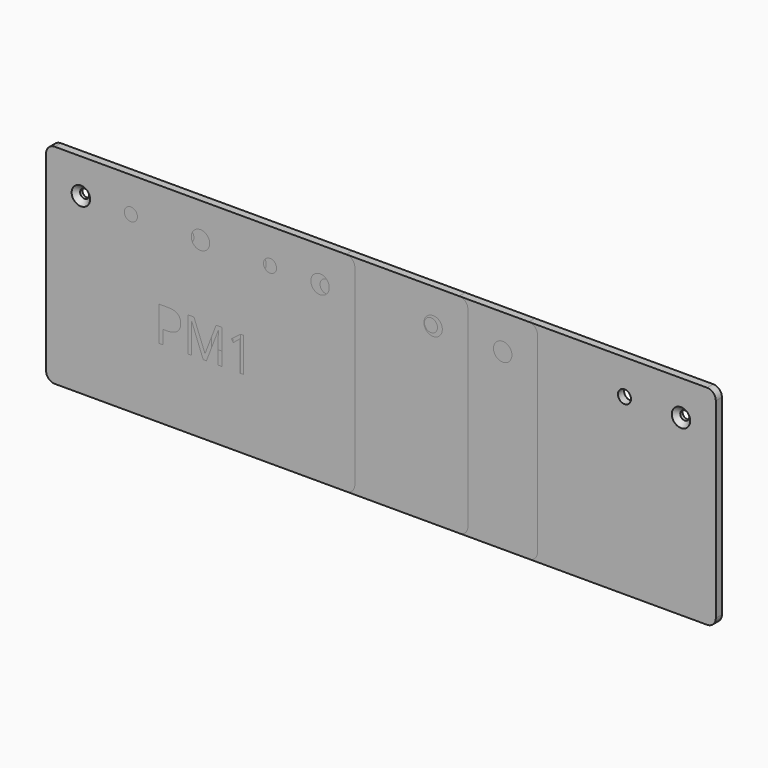
from build123d import *

# Parameters (mm, degrees)
F1_W            = 488.95
F1_H            = 152.4
F2_DEPTH        = 5.588
F3_D            = 9.525
F4_D            = 6.6
F4_CSINK_D      = 13.44
F4_CSINK_ANGLE  = 90
F5_R            = 6.35
F6_W            = 358.775
F6_H            = 152.4
F7_DEPTH        = 5.588
F8_R            = 6.35
F9_D            = 9.525
F10_D           = 6.6
F10_CSINK_D     = 13.44
F10_CSINK_ANGLE = 90
F11_W           = 307.975
F11_H           = 152.4
F12_DEPTH       = 5.588
F13_R           = 6.35
F14_D           = 9.525
F15_D           = 6.6
F15_CSINK_D     = 13.44
F15_CSINK_ANGLE = 90
F16_W           = 225.425
F16_H           = 152.4
F17_DEPTH       = 5.588
F18_R           = 6.35
F19_D           = 6.6
F19_CSINK_D     = 13.44
F19_CSINK_ANGLE = 90
F20_D           = 9.525


# Not quite as in the source:
# - a variable given as a bare number and used for a length is read in inches; the dataset says mm whatever the document's units were
# - a length typed as a fraction of an inch, garbled in the dataset ("3 / 203.2 mm" for 3/8 in), is restored


with BuildPart() as f2:
    # F1 (on Front) → F2 (new body)
    with BuildSketch(Plane.XZ):
        with Locations((244.475, -76.2)):
            Rectangle(F1_W, F1_H)
        with BuildLine():
            add(Edge.make_bspline(
                [(217.0492838542, -76.4149739583), (226.4860894097, -76.4149739583), (226.4860894097, -83.7516493056)],
                knots=[0, 0, 0, 1, 1, 1], degree=2))
            add(Edge.make_bspline(
                [(226.4860894097, -83.7516493056), (226.4860894097, -87.5770833333), (223.8760850694, -89.6358723958)],
                knots=[0, 0, 0, 1, 1, 1], degree=2))
            add(Edge.make_bspline(
                [(223.8760850694, -89.6358723958), (221.2660807292, -91.6946614583), (216.4098741319, -91.6946614583)],
                knots=[0, 0, 0, 1, 1, 1], degree=2))
            Line((216.4098741319, -91.6946614583), (213.4443359375, -91.6946614583))
            Line((213.4443359375, -91.6946614583), (213.4443359375, -101.6))
            Line((213.4443359375, -101.6), (210.5173828125, -101.6))
            Line((210.5173828125, -101.6), (210.5173828125, -76.4149739583))
            Line((210.5173828125, -76.4149739583), (217.0492838542, -76.4149739583))
        make_face(mode=Mode.SUBTRACT)
        with BuildLine():
            Line((245.2604817708, -101.6), (242.9012803819, -101.6))
            Line((242.9012803819, -101.6), (234.3574435764, -79.27578125))
            Line((234.3574435764, -79.27578125), (234.2196397569, -79.27578125))
            add(Edge.make_bspline(
                [(234.2196397569, -79.27578125), (234.4621744792, -81.9271267361), (234.4621744792, -85.5816840278)],
                knots=[0, 0, 0, 1, 1, 1], degree=2))
            Line((234.4621744792, -85.5816840278), (234.4621744792, -101.6))
            Line((234.4621744792, -101.6), (231.7557074653, -101.6))
            Line((231.7557074653, -101.6), (231.7557074653, -76.4149739583))
            Line((231.7557074653, -76.4149739583), (236.1654296875, -76.4149739583))
            Line((236.1654296875, -76.4149739583), (244.1415147569, -97.1902777778))
            Line((244.1415147569, -97.1902777778), (244.2793185764, -97.1902777778))
            Line((244.2793185764, -97.1902777778), (252.3215494792, -76.4149739583))
            Line((252.3215494792, -76.4149739583), (256.6981987847, -76.4149739583))
            Line((256.6981987847, -76.4149739583), (256.6981987847, -101.6))
            Line((256.6981987847, -101.6), (253.7712456597, -101.6))
            Line((253.7712456597, -101.6), (253.7712456597, -85.3722222222))
            add(Edge.make_bspline(
                [(253.7712456597, -85.3722222222), (253.7712456597, -82.5830729167), (254.0137803819, -79.3088541667)],
                knots=[0, 0, 0, 1, 1, 1], degree=2))
            Line((254.0137803819, -79.3088541667), (253.8759765625, -79.3088541667))
            Line((253.8759765625, -79.3088541667), (245.2604817708, -101.6))
        make_face(mode=Mode.SUBTRACT)
        Polygon((279.6067057292, -93.2105034722), (279.6067057292, -95.8122395833), (275.8694661458, -95.8122395833), (275.8694661458, -101.6), (273.1299262153, -101.6), (273.1299262153, -95.8122395833), (260.8819227431, -95.8122395833), (260.8819227431, -93.315234375), (272.8377821181, -76.2771701389), (275.8694661458, -76.2771701389), (275.8694661458, -93.2105034722), align=None, mode=Mode.SUBTRACT)
    extrude(amount=-F2_DEPTH)

    # F3 (through all)
    with Locations(Plane.XZ):
        with Locations((66.675, -25.4), (422.275, -25.4)):
            Hole(F3_D / 2)

    # F4 (through all)
    with Locations(Plane.XZ):
        with Locations((25.4, -25.4), (463.55, -25.4), (311.15, -25.4), (177.8, -25.4)):
            CounterSinkHole(F4_D / 2, F4_CSINK_D / 2, counter_sink_angle=F4_CSINK_ANGLE)

    # F5
    f5_edges = [f2.edges().sort_by_distance(p)[0] for p in [
        (0, 2.794, 0),
        (488.95, 2.794, 0),
        (488.95, 2.794, -152.4),
        (0, 2.794, -152.4),
    ]]
    fillet(f5_edges, radius=F5_R)


with BuildPart() as f7:
    # F6 (on Front) → F7 (new body)
    with BuildSketch(Plane.XZ):
        with Locations((179.3875, -76.2)):
            Rectangle(F6_W, F6_H)
        with BuildLine():
            add(Edge.make_bspline(
                [(152.6425347222, -76.4149739583), (162.0793402778, -76.4149739583), (162.0793402778, -83.7516493056)],
                knots=[0, 0, 0, 1, 1, 1], degree=2))
            add(Edge.make_bspline(
                [(162.0793402778, -83.7516493056), (162.0793402778, -87.5770833333), (159.4693359375, -89.6358723958)],
                knots=[0, 0, 0, 1, 1, 1], degree=2))
            add(Edge.make_bspline(
                [(159.4693359375, -89.6358723958), (156.8593315972, -91.6946614583), (152.003125, -91.6946614583)],
                knots=[0, 0, 0, 1, 1, 1], degree=2))
            Line((152.003125, -91.6946614583), (149.0375868056, -91.6946614583))
            Line((149.0375868056, -91.6946614583), (149.0375868056, -101.6))
            Line((149.0375868056, -101.6), (146.1106336806, -101.6))
            Line((146.1106336806, -101.6), (146.1106336806, -76.4149739583))
            Line((146.1106336806, -76.4149739583), (152.6425347222, -76.4149739583))
        make_face(mode=Mode.SUBTRACT)
        with BuildLine():
            Line((180.8537326389, -101.6), (178.49453125, -101.6))
            Line((178.49453125, -101.6), (169.9506944444, -79.27578125))
            Line((169.9506944444, -79.27578125), (169.812890625, -79.27578125))
            add(Edge.make_bspline(
                [(169.812890625, -79.27578125), (170.0554253472, -81.9271267361), (170.0554253472, -85.5816840278)],
                knots=[0, 0, 0, 1, 1, 1], degree=2))
            Line((170.0554253472, -85.5816840278), (170.0554253472, -101.6))
            Line((170.0554253472, -101.6), (167.3489583333, -101.6))
            Line((167.3489583333, -101.6), (167.3489583333, -76.4149739583))
            Line((167.3489583333, -76.4149739583), (171.7586805556, -76.4149739583))
            Line((171.7586805556, -76.4149739583), (179.734765625, -97.1902777778))
            Line((179.734765625, -97.1902777778), (179.8725694444, -97.1902777778))
            Line((179.8725694444, -97.1902777778), (187.9148003472, -76.4149739583))
            Line((187.9148003472, -76.4149739583), (192.2914496528, -76.4149739583))
            Line((192.2914496528, -76.4149739583), (192.2914496528, -101.6))
            Line((192.2914496528, -101.6), (189.3644965278, -101.6))
            Line((189.3644965278, -101.6), (189.3644965278, -85.3722222222))
            add(Edge.make_bspline(
                [(189.3644965278, -85.3722222222), (189.3644965278, -82.5830729167), (189.60703125, -79.3088541667)],
                knots=[0, 0, 0, 1, 1, 1], degree=2))
            Line((189.60703125, -79.3088541667), (189.4692274306, -79.3088541667))
            Line((189.4692274306, -79.3088541667), (180.8537326389, -101.6))
        make_face(mode=Mode.SUBTRACT)
        with BuildLine():
            add(Edge.make_bspline(
                [(211.0327690972, -77.7351345486), (213.0667534722, -79.4135850694), (213.0667534722, -82.3405381944)],
                knots=[0, 0, 0, 1, 1, 1], degree=2))
            add(Edge.make_bspline(
                [(213.0667534722, -82.3405381944), (213.0667534722, -84.7548611111), (211.7135199653, -86.2872395833)],
                knots=[0, 0, 0, 1, 1, 1], degree=2))
            add(Edge.make_bspline(
                [(211.7135199653, -86.2872395833), (210.3602864583, -87.8196180556), (207.8798177083, -88.3377604167)],
                knots=[0, 0, 0, 1, 1, 1], degree=2))
            Line((207.8798177083, -88.3377604167), (207.8798177083, -88.4755642361))
            add(Edge.make_bspline(
                [(207.8798177083, -88.4755642361), (210.9115017361, -88.850390625), (212.3749782986, -90.4020616319)],
                knots=[0, 0, 0, 1, 1, 1], degree=2))
            add(Edge.make_bspline(
                [(212.3749782986, -90.4020616319), (213.8384548611, -91.9537326389), (213.8384548611, -94.4672743056)],
                knots=[0, 0, 0, 1, 1, 1], degree=2))
            add(Edge.make_bspline(
                [(213.8384548611, -94.4672743056), (213.8384548611, -98.0667100694), (211.3414496528, -100.0069878472)],
                knots=[0, 0, 0, 1, 1, 1], degree=2))
            add(Edge.make_bspline(
                [(211.3414496528, -100.0069878472), (208.8444444444, -101.947265625), (204.2473090278, -101.947265625)],
                knots=[0, 0, 0, 1, 1, 1], degree=2))
            add(Edge.make_bspline(
                [(204.2473090278, -101.947265625), (202.2463975694, -101.947265625), (200.5844835069, -101.6440972222)],
                knots=[0, 0, 0, 1, 1, 1], degree=2))
            add(Edge.make_bspline(
                [(200.5844835069, -101.6440972222), (198.9225694444, -101.3409288194), (197.3571180556, -100.5857638889)],
                knots=[0, 0, 0, 1, 1, 1], degree=2))
            Line((197.3571180556, -100.5857638889), (197.3571180556, -97.8627604167))
            add(Edge.make_bspline(
                [(197.3571180556, -97.8627604167), (198.9942274306, -98.673046875), (200.8463107639, -99.0947265625)],
                knots=[0, 0, 0, 1, 1, 1], degree=2))
            add(Edge.make_bspline(
                [(200.8463107639, -99.0947265625), (202.6983940972, -99.51640625), (204.3520399306, -99.51640625)],
                knots=[0, 0, 0, 1, 1, 1], degree=2))
            add(Edge.make_bspline(
                [(204.3520399306, -99.51640625), (210.8784288194, -99.51640625), (210.8784288194, -94.4011284722)],
                knots=[0, 0, 0, 1, 1, 1], degree=2))
            add(Edge.make_bspline(
                [(210.8784288194, -94.4011284722), (210.8784288194, -89.8150173611), (203.6795572917, -89.8150173611)],
                knots=[0, 0, 0, 1, 1, 1], degree=2))
            Line((203.6795572917, -89.8150173611), (201.1990885417, -89.8150173611))
            Line((201.1990885417, -89.8150173611), (201.1990885417, -87.3565972222))
            Line((201.1990885417, -87.3565972222), (203.7126302083, -87.3565972222))
            add(Edge.make_bspline(
                [(203.7126302083, -87.3565972222), (206.6561197917, -87.3565972222), (208.3786675347, -86.0557291667)],
                knots=[0, 0, 0, 1, 1, 1], degree=2))
            add(Edge.make_bspline(
                [(208.3786675347, -86.0557291667), (210.1012152778, -84.7548611111), (210.1012152778, -82.4452690972)],
                knots=[0, 0, 0, 1, 1, 1], degree=2))
            add(Edge.make_bspline(
                [(210.1012152778, -82.4452690972), (210.1012152778, -80.6042100694), (208.8361762153, -79.5513888889)],
                knots=[0, 0, 0, 1, 1, 1], degree=2))
            add(Edge.make_bspline(
                [(208.8361762153, -79.5513888889), (207.5711371528, -78.4985677083), (205.3993489583, -78.4985677083)],
                knots=[0, 0, 0, 1, 1, 1], degree=2))
            add(Edge.make_bspline(
                [(205.3993489583, -78.4985677083), (203.745703125, -78.4985677083), (202.2822265625, -78.9478081597)],
                knots=[0, 0, 0, 1, 1, 1], degree=2))
            add(Edge.make_bspline(
                [(202.2822265625, -78.9478081597), (200.81875, -79.3970486111), (198.9391059028, -80.6042100694)],
                knots=[0, 0, 0, 1, 1, 1], degree=2))
            Line((198.9391059028, -80.6042100694), (197.494921875, -78.6749565972))
            add(Edge.make_bspline(
                [(197.494921875, -78.6749565972), (199.0438368056, -77.4512586806), (201.066796875, -76.7539713542)],
                knots=[0, 0, 0, 1, 1, 1], degree=2))
            add(Edge.make_bspline(
                [(201.066796875, -76.7539713542), (203.0897569444, -76.0566840278), (205.333203125, -76.0566840278)],
                knots=[0, 0, 0, 1, 1, 1], degree=2))
            add(Edge.make_bspline(
                [(205.333203125, -76.0566840278), (208.9987847222, -76.0566840278), (211.0327690972, -77.7351345486)],
                knots=[0, 0, 0, 1, 1, 1], degree=2))
        make_face(mode=Mode.SUBTRACT)
    extrude(amount=-F7_DEPTH)

    # F8
    f8_edges = [f7.edges().sort_by_distance(p)[0] for p in [
        (0, 2.794, 0),
        (358.775, 2.794, 0),
        (358.775, 2.794, -152.4),
        (0, 2.794, -152.4),
    ]]
    fillet(f8_edges, radius=F8_R)

    # F9 (through all)
    with Locations(Plane.XZ):
        with Locations((280.9875, -25.4), (77.7875, -25.4)):
            Hole(F9_D / 2)

    # F10 (through all)
    with Locations(Plane.XZ):
        with Locations((25.4, -25.4), (179.3875, -25.4), (333.375, -25.4)):
            CounterSinkHole(F10_D / 2, F10_CSINK_D / 2, counter_sink_angle=F10_CSINK_ANGLE)


with BuildPart() as f12:
    # F11 (on Front) → F12 (new body)
    with BuildSketch(Plane.XZ):
        with Locations((153.9875, -76.2)):
            Rectangle(F11_W, F11_H)
        with BuildLine():
            add(Edge.make_bspline(
                [(127.1543402778, -76.4149739583), (136.5911458333, -76.4149739583), (136.5911458333, -83.7516493056)],
                knots=[0, 0, 0, 1, 1, 1], degree=2))
            add(Edge.make_bspline(
                [(136.5911458333, -83.7516493056), (136.5911458333, -87.5770833333), (133.9811414931, -89.6358723958)],
                knots=[0, 0, 0, 1, 1, 1], degree=2))
            add(Edge.make_bspline(
                [(133.9811414931, -89.6358723958), (131.3711371528, -91.6946614583), (126.5149305556, -91.6946614583)],
                knots=[0, 0, 0, 1, 1, 1], degree=2))
            Line((126.5149305556, -91.6946614583), (123.5493923611, -91.6946614583))
            Line((123.5493923611, -91.6946614583), (123.5493923611, -101.6))
            Line((123.5493923611, -101.6), (120.6224392361, -101.6))
            Line((120.6224392361, -101.6), (120.6224392361, -76.4149739583))
            Line((120.6224392361, -76.4149739583), (127.1543402778, -76.4149739583))
        make_face(mode=Mode.SUBTRACT)
        with BuildLine():
            Line((155.3655381944, -101.6), (153.0063368056, -101.6))
            Line((153.0063368056, -101.6), (144.4625, -79.27578125))
            Line((144.4625, -79.27578125), (144.3246961806, -79.27578125))
            add(Edge.make_bspline(
                [(144.3246961806, -79.27578125), (144.5672309028, -81.9271267361), (144.5672309028, -85.5816840278)],
                knots=[0, 0, 0, 1, 1, 1], degree=2))
            Line((144.5672309028, -85.5816840278), (144.5672309028, -101.6))
            Line((144.5672309028, -101.6), (141.8607638889, -101.6))
            Line((141.8607638889, -101.6), (141.8607638889, -76.4149739583))
            Line((141.8607638889, -76.4149739583), (146.2704861111, -76.4149739583))
            Line((146.2704861111, -76.4149739583), (154.2465711806, -97.1902777778))
            Line((154.2465711806, -97.1902777778), (154.384375, -97.1902777778))
            Line((154.384375, -97.1902777778), (162.4266059028, -76.4149739583))
            Line((162.4266059028, -76.4149739583), (166.8032552083, -76.4149739583))
            Line((166.8032552083, -76.4149739583), (166.8032552083, -101.6))
            Line((166.8032552083, -101.6), (163.8763020833, -101.6))
            Line((163.8763020833, -101.6), (163.8763020833, -85.3722222222))
            add(Edge.make_bspline(
                [(163.8763020833, -85.3722222222), (163.8763020833, -82.5830729167), (164.1188368056, -79.3088541667)],
                knots=[0, 0, 0, 1, 1, 1], degree=2))
            Line((164.1188368056, -79.3088541667), (163.9810329861, -79.3088541667))
            Line((163.9810329861, -79.3088541667), (155.3655381944, -101.6))
        make_face(mode=Mode.SUBTRACT)
        with BuildLine():
            Line((188.5266493056, -98.9486545139), (188.5266493056, -101.6))
            Line((188.5266493056, -101.6), (171.9736545139, -101.6))
            Line((171.9736545139, -101.6), (171.9736545139, -99.1360677083))
            Line((171.9736545139, -99.1360677083), (178.6047743056, -92.471875))
            add(Edge.make_bspline(
                [(178.6047743056, -92.471875), (181.6364583333, -89.4016059028), (182.6010850694, -88.0924696181)],
                knots=[0, 0, 0, 1, 1, 1], degree=2))
            add(Edge.make_bspline(
                [(182.6010850694, -88.0924696181), (183.5657118056, -86.7833333333), (184.0480251736, -85.5430989583)],
                knots=[0, 0, 0, 1, 1, 1], degree=2))
            add(Edge.make_bspline(
                [(184.0480251736, -85.5430989583), (184.5303385417, -84.3028645833), (184.5303385417, -82.8752170139)],
                knots=[0, 0, 0, 1, 1, 1], degree=2))
            add(Edge.make_bspline(
                [(184.5303385417, -82.8752170139), (184.5303385417, -80.8577690972), (183.306640625, -79.6781684028)],
                knots=[0, 0, 0, 1, 1, 1], degree=2))
            add(Edge.make_bspline(
                [(183.306640625, -79.6781684028), (182.0829427083, -78.4985677083), (179.9111545139, -78.4985677083)],
                knots=[0, 0, 0, 1, 1, 1], degree=2))
            add(Edge.make_bspline(
                [(179.9111545139, -78.4985677083), (178.345703125, -78.4985677083), (176.9401041667, -79.0167100694)],
                knots=[0, 0, 0, 1, 1, 1], degree=2))
            add(Edge.make_bspline(
                [(176.9401041667, -79.0167100694), (175.5345052083, -79.5348524306), (173.8147135417, -80.8963541667)],
                knots=[0, 0, 0, 1, 1, 1], degree=2))
            Line((173.8147135417, -80.8963541667), (172.2988715278, -78.9505642361))
            add(Edge.make_bspline(
                [(172.2988715278, -78.9505642361), (175.7770399306, -76.0566840278), (179.8780815972, -76.0566840278)],
                knots=[0, 0, 0, 1, 1, 1], degree=2))
            add(Edge.make_bspline(
                [(179.8780815972, -76.0566840278), (183.4279079861, -76.0566840278), (185.4425998264, -77.8729383681)],
                knots=[0, 0, 0, 1, 1, 1], degree=2))
            add(Edge.make_bspline(
                [(185.4425998264, -77.8729383681), (187.4572916667, -79.6891927083), (187.4572916667, -82.7539496528)],
                knots=[0, 0, 0, 1, 1, 1], degree=2))
            add(Edge.make_bspline(
                [(187.4572916667, -82.7539496528), (187.4572916667, -85.1517361111), (186.1123263889, -87.4944010417)],
                knots=[0, 0, 0, 1, 1, 1], degree=2))
            add(Edge.make_bspline(
                [(186.1123263889, -87.4944010417), (184.7673611111, -89.8370659722), (181.0852430556, -93.4199652778)],
                knots=[0, 0, 0, 1, 1, 1], degree=2))
            Line((181.0852430556, -93.4199652778), (175.5730902778, -98.8108506944))
            Line((175.5730902778, -98.8108506944), (175.5730902778, -98.9486545139))
            Line((175.5730902778, -98.9486545139), (188.5266493056, -98.9486545139))
        make_face(mode=Mode.SUBTRACT)
    extrude(amount=-F12_DEPTH)

    # F13
    f13_edges = [f12.edges().sort_by_distance(p)[0] for p in [
        (0, 2.794, 0),
        (307.975, 2.794, 0),
        (307.975, 2.794, -152.4),
        (0, 2.794, -152.4),
    ]]
    fillet(f13_edges, radius=F13_R)

    # F14 (through all)
    with Locations(Plane.XZ):
        with Locations((204.7875, -25.4), (103.1875, -25.4)):
            Hole(F14_D / 2)

    # F15 (through all)
    with Locations(Plane.XZ):
        with Locations((25.4, -25.4), (153.9875, -25.4), (282.575, -25.4)):
            CounterSinkHole(F15_D / 2, F15_CSINK_D / 2, counter_sink_angle=F15_CSINK_ANGLE)


with BuildPart() as f17:
    # F16 (on Front) → F17 (new body)
    with BuildSketch(Plane.XZ):
        with Locations((112.7125, -76.2)):
            Rectangle(F16_W, F16_H)
        with BuildLine():
            add(Edge.make_bspline(
                [(88.8614149306, -76.4149739583), (98.2982204861, -76.4149739583), (98.2982204861, -83.7516493056)],
                knots=[0, 0, 0, 1, 1, 1], degree=2))
            add(Edge.make_bspline(
                [(98.2982204861, -83.7516493056), (98.2982204861, -87.5770833333), (95.6882161458, -89.6358723958)],
                knots=[0, 0, 0, 1, 1, 1], degree=2))
            add(Edge.make_bspline(
                [(95.6882161458, -89.6358723958), (93.0782118056, -91.6946614583), (88.2220052083, -91.6946614583)],
                knots=[0, 0, 0, 1, 1, 1], degree=2))
            Line((88.2220052083, -91.6946614583), (85.2564670139, -91.6946614583))
            Line((85.2564670139, -91.6946614583), (85.2564670139, -101.6))
            Line((85.2564670139, -101.6), (82.3295138889, -101.6))
            Line((82.3295138889, -101.6), (82.3295138889, -76.4149739583))
            Line((82.3295138889, -76.4149739583), (88.8614149306, -76.4149739583))
        make_face(mode=Mode.SUBTRACT)
        with BuildLine():
            Line((117.0726128472, -101.6), (114.7134114583, -101.6))
            Line((114.7134114583, -101.6), (106.1695746528, -79.27578125))
            Line((106.1695746528, -79.27578125), (106.0317708333, -79.27578125))
            add(Edge.make_bspline(
                [(106.0317708333, -79.27578125), (106.2743055556, -81.9271267361), (106.2743055556, -85.5816840278)],
                knots=[0, 0, 0, 1, 1, 1], degree=2))
            Line((106.2743055556, -85.5816840278), (106.2743055556, -101.6))
            Line((106.2743055556, -101.6), (103.5678385417, -101.6))
            Line((103.5678385417, -101.6), (103.5678385417, -76.4149739583))
            Line((103.5678385417, -76.4149739583), (107.9775607639, -76.4149739583))
            Line((107.9775607639, -76.4149739583), (115.9536458333, -97.1902777778))
            Line((115.9536458333, -97.1902777778), (116.0914496528, -97.1902777778))
            Line((116.0914496528, -97.1902777778), (124.1336805556, -76.4149739583))
            Line((124.1336805556, -76.4149739583), (128.5103298611, -76.4149739583))
            Line((128.5103298611, -76.4149739583), (128.5103298611, -101.6))
            Line((128.5103298611, -101.6), (125.5833767361, -101.6))
            Line((125.5833767361, -101.6), (125.5833767361, -85.3722222222))
            add(Edge.make_bspline(
                [(125.5833767361, -85.3722222222), (125.5833767361, -82.5830729167), (125.8259114583, -79.3088541667)],
                knots=[0, 0, 0, 1, 1, 1], degree=2))
            Line((125.8259114583, -79.3088541667), (125.6881076389, -79.3088541667))
            Line((125.6881076389, -79.3088541667), (117.0726128472, -101.6))
        make_face(mode=Mode.SUBTRACT)
        with BuildLine():
            Line((144.2695746528, -76.4149739583), (144.2695746528, -101.6))
            Line((144.2695746528, -101.6), (141.4804253472, -101.6))
            Line((141.4804253472, -101.6), (141.4804253472, -83.6524305556))
            add(Edge.make_bspline(
                [(141.4804253472, -83.6524305556), (141.4804253472, -81.408984375), (141.6182291667, -79.4135850694)],
                knots=[0, 0, 0, 1, 1, 1], degree=2))
            add(Edge.make_bspline(
                [(141.6182291667, -79.4135850694), (141.2599392361, -79.7773871528), (140.8106987847, -80.1715060764)],
                knots=[0, 0, 0, 1, 1, 1], degree=2))
            add(Edge.make_bspline(
                [(140.8106987847, -80.1715060764), (140.3614583333, -80.565625), (136.7124131944, -83.5311631944)],
                knots=[0, 0, 0, 1, 1, 1], degree=2))
            Line((136.7124131944, -83.5311631944), (135.1965711806, -81.5688368056))
            Line((135.1965711806, -81.5688368056), (141.8607638889, -76.4149739583))
            Line((141.8607638889, -76.4149739583), (144.2695746528, -76.4149739583))
        make_face(mode=Mode.SUBTRACT)
    extrude(amount=-F17_DEPTH)

    # F18
    f18_edges = [f17.edges().sort_by_distance(p)[0] for p in [
        (0, 2.794, 0),
        (225.425, 2.794, 0),
        (225.425, 2.794, -152.4),
        (0, 2.794, -152.4),
    ]]
    fillet(f18_edges, radius=F18_R)

    # F19 (through all)
    with Locations(Plane.XZ):
        with Locations((25.4, -25.4), (112.7125, -25.4), (200.025, -25.4)):
            CounterSinkHole(F19_D / 2, F19_CSINK_D / 2, counter_sink_angle=F19_CSINK_ANGLE)

    # F20 (through all)
    with Locations(Plane.XZ):
        with Locations((163.5125, -25.4), (61.9125, -25.4)):
            Hole(F20_D / 2)


solid = Compound([f2.part, f7.part, f12.part, f17.part])
